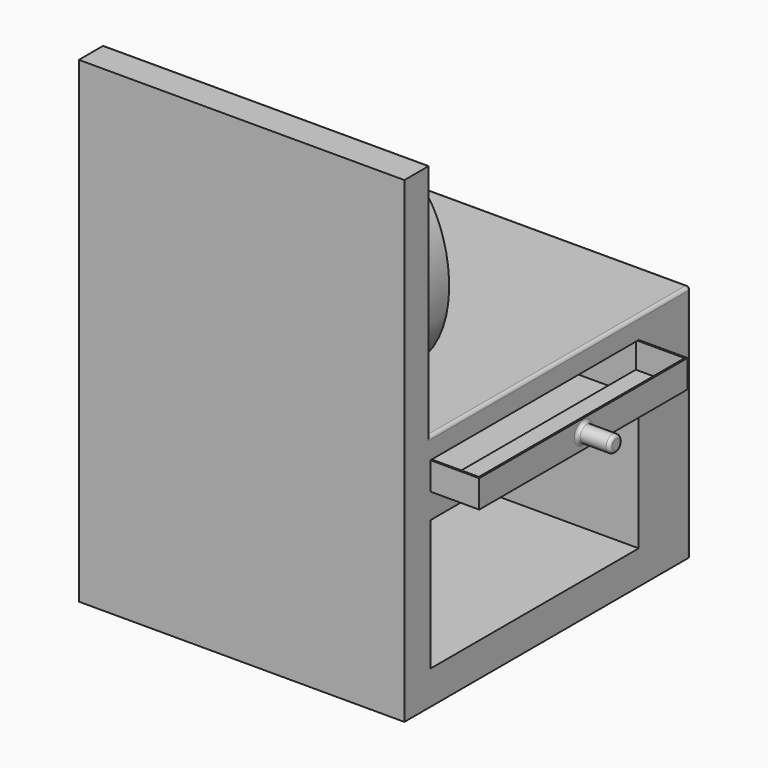
from build123d import *

# Parameters (mm, degrees)
F0_W         = 406.4
F0_H         = 203.9072960615
F1_DEPTH     = 508
F3_DEPTH     = 66.04
F4_W         = 101.6
F4_H         = 123.825
F5_DEPTH     = 88.9
F6_W         = 406.4
F6_H         = 43.1739762425
F7_DEPTH     = 76.2
F8_T         = 2.54
F8_T3_DEPTH  = 513.08
F8_T5_DEPTH  = 48.2539762425
F8_T7_DEPTH  = 411.48
F8_T9_DEPTH  = 93.98
F8_T11_DEPTH = 106.68
F8_T13_DEPTH = 128.905
F8_T15_DEPTH = 106.68
F8_T17_DEPTH = 106.68
F9_R         = 12.7
F10_DEPTH    = 50.8
F11_R        = 5.08


# Not quite as in the source:
# - a shell that OpenCascade refuses in one call is made with other operations: the cavity is built on its own and cut out


with BuildPart() as f1:
    # F0 (on Right) → F1 (new body)
    with BuildSketch(Plane.YZ):
        Polygon((-406.4, 487.9180668924), (-457.2, 487.9180668924), (-457.2, -256.5294758297), (-406.4, -256.5294758297), (0, -256.5294758297), (101.6, -256.5294758297), (101.6, 115.6942955313), (-406.4, 115.6942955313), align=None)
        with Locations((-203.2, -101.9536480308)):
            Rectangle(F0_W, F0_H, mode=Mode.SUBTRACT)
    extrude(amount=F1_DEPTH)

    # F4 (on face) → F5 (cut)
    with BuildSketch(Plane(origin=(0, 101.6, 0), x_dir=(-1, 0, 0), z_dir=(0, 1, 0))):
        with Locations((-434.9174816871, -150.9387567639)):
            Rectangle(F4_W, F4_H)
        with Locations((-258.955590483, -150.9387567639)):
            Rectangle(F4_W, F4_H)
        with Locations((-82.984390483, -150.9387567639)):
            Rectangle(F4_W, F4_H)
    extrude(amount=-F5_DEPTH, mode=Mode.SUBTRACT)

    # F6 (on face) → F7 (join)
    with BuildSketch(Plane.YZ.offset(508)):
        with Locations((-203.2, 60.8287490904)):
            Rectangle(F6_W, F6_H)
    extrude(amount=F7_DEPTH)

    # F8: shell of thickness 2.54, made by hand


with BuildPart() as f3:
    # F2 (on face) → F3 (new body)
    with BuildSketch(Plane(origin=(0, -406.4, 0), x_dir=(-1, 0, 0), z_dir=(0, 1, 0))):
        with BuildLine():
            add(Edge.make_bspline(
                [(-288.5718345642, 419.7029471397), (-347.6021943127, 419.1585833452), (-459.5465679813, 479.02511134), (-545.5014679601, 101.5749100376), (9.3815956545, 69.448257945), (-42.615563951, 501.5186421954), (-218.7578993917, 420.3467544759), (-288.5718345642, 419.7029471397)],
                knots=[0, 0, 0, 0, 0.1571960663, 0.3561031036, 0.6066974638, 0.8140875979, 1, 1, 1, 1], degree=3))
        make_face()
    extrude(amount=F3_DEPTH)


with BuildPart() as f8_core1:
    # F8_t2: copy of F1
    add(f1.part)

    # the walls: a layer under each face that stays
    f8_faces = [f8_core1.faces().sort_by_distance(p)[0] for p in [
        (254, -152.4, 115.6942955313),
        (254, 101.6, -70.4175901492),
        (254, -406.4, 301.8061812119),
        (0, 8.4666666667, -132.454885376),
        (508, 8.4666666667, -132.454885376),
        (254, -177.8, -256.5294758297),
        (258.955590483, 57.15, -212.8512567639),
        (309.755590483, 57.15, -150.9387567639),
        (258.955590483, 57.15, -89.0262567639),
        (208.155590483, 57.15, -150.9387567639),
        (485.7174816871, 57.15, -150.9387567639),
        (434.9174816871, 57.15, -89.0262567639),
        (384.1174816871, 57.15, -150.9387567639),
        (434.9174816871, 57.15, -212.8512567639),
        (82.984390483, 57.15, -212.8512567639),
        (133.784390483, 57.15, -150.9387567639),
        (82.984390483, 57.15, -89.0262567639),
        (32.184390483, 57.15, -150.9387567639),
        (254, -431.8, 487.9180668924),
        (254, -457.2, 115.6942955313),
        (254, -406.4, -101.9536480308),
        (254, -203.2, 0),
        (254, 0, -101.9536480308),
        (254, -203.2, -203.9072960615),
        (546.1, -406.4, 60.8287490904),
        (546.1, -203.2, 39.2417609692),
        (546.1, 0, 60.8287490904),
        (258.955590483, 12.7, -150.9387567639),
        (434.9174816871, 12.7, -150.9387567639),
        (82.984390483, 12.7, -150.9387567639),
        (584.2, -203.2, 60.8287490904),
    ]]
    thicken(f8_faces, amount=-F8_T, mode=Mode.SUBTRACT)

    # F8_s4 → F8_t3 (cut)
    with BuildSketch(Plane.YZ.offset(-2.54)):
        Polygon((-406.3746, 115.7196955313), (-406.4, 113.1542955313), (-408.94, 113.1542955313), (-408.94, 115.6942955313), align=None)
        Polygon((-406.3746, -203.8818960615), (-408.94, -203.9072960615), (-408.94, -206.4472960615), (-406.4, -206.4472960615), align=None)
        Polygon((-406.3746, -0.0254), (-408.94, 0), (-408.94, 2.54), (-406.4, 2.54), align=None)
        Polygon((-0.0254, -0.0254), (0, 2.54), (2.54, 2.54), (2.54, 0), align=None)
        Polygon((-0.0254, -203.8818960615), (2.54, -203.9072960615), (2.54, -206.4472960615), (0, -206.4472960615), align=None)
    extrude(amount=F8_T3_DEPTH, mode=Mode.SUBTRACT)

    # F8_s6 → F8_t5 (cut)
    with BuildSketch(Plane.XY.offset(36.7017609692)):
        Polygon((508.0254, -406.4254), (505.46, -406.4), (505.46, -403.86), (508, -403.86), align=None)
        Polygon((508.0254, 0.0254), (505.46, 0), (505.46, -2.54), (508, -2.54), align=None)
    extrude(amount=F8_T5_DEPTH, mode=Mode.SUBTRACT)

    # F8_s8 → F8_t7 (cut)
    with BuildSketch(Plane.XZ.offset(-2.54)):
        Polygon((508.0254, 39.2163609692), (505.46, 39.2417609692), (505.46, 41.7817609692), (508, 41.7817609692), align=None)
    extrude(amount=F8_T7_DEPTH, mode=Mode.SUBTRACT)

    # F8_s10 → F8_t9 (cut)
    with BuildSketch(Plane.XZ.offset(-104.14)):
        Polygon((309.730190483, -212.8258567639), (309.755590483, -215.3912567639), (312.295590483, -215.3912567639), (312.295590483, -212.8512567639), align=None)
        Polygon((208.180990483, -212.8258567639), (208.155590483, -215.3912567639), (205.615590483, -215.3912567639), (205.615590483, -212.8512567639), align=None)
        Polygon((309.730190483, -89.0516567639), (312.295590483, -89.0262567639), (312.295590483, -86.4862567639), (309.755590483, -86.4862567639), align=None)
        Polygon((208.180990483, -89.0516567639), (208.155590483, -86.4862567639), (205.615590483, -86.4862567639), (205.615590483, -89.0262567639), align=None)
        Polygon((485.6920816871, -89.0516567639), (488.2574816871, -89.0262567639), (488.2574816871, -86.4862567639), (485.7174816871, -86.4862567639), align=None)
        Polygon((485.6920816871, -212.8258567639), (488.2574816871, -212.8512567639), (488.2574816871, -215.3912567639), (485.7174816871, -215.3912567639), align=None)
        Polygon((384.1428816871, -89.0516567639), (384.1174816871, -86.4862567639), (381.5774816871, -86.4862567639), (381.5774816871, -89.0262567639), align=None)
        Polygon((384.1428816871, -212.8258567639), (381.5774816871, -212.8512567639), (381.5774816871, -215.3912567639), (384.1174816871, -215.3912567639), align=None)
        Polygon((133.758990483, -212.8258567639), (133.784390483, -215.3912567639), (136.324390483, -215.3912567639), (136.324390483, -212.8512567639), align=None)
        Polygon((32.209790483, -212.8258567639), (32.184390483, -215.3912567639), (29.644390483, -215.3912567639), (29.644390483, -212.8512567639), align=None)
        Polygon((133.758990483, -89.0516567639), (136.324390483, -89.0262567639), (136.324390483, -86.4862567639), (133.784390483, -86.4862567639), align=None)
        Polygon((32.209790483, -89.0516567639), (32.184390483, -86.4862567639), (29.644390483, -86.4862567639), (29.644390483, -89.0262567639), align=None)
    extrude(amount=F8_T9_DEPTH, mode=Mode.SUBTRACT)

    # F8_s12 → F8_t11 (cut)
    with BuildSketch(Plane.YZ.offset(205.615590483)):
        Polygon((12.7254, -212.8258567639), (12.7, -215.3912567639), (10.16, -215.3912567639), (10.16, -212.8512567639), align=None)
        Polygon((12.7254, -89.0516567639), (12.7, -86.4862567639), (10.16, -86.4862567639), (10.16, -89.0262567639), align=None)
    extrude(amount=F8_T11_DEPTH, mode=Mode.SUBTRACT)

    # F8_s14 → F8_t13 (cut)
    with BuildSketch(Plane.XY.offset(-215.3912567639)):
        Polygon((309.730190483, 12.7254), (312.295590483, 12.7), (312.295590483, 10.16), (309.755590483, 10.16), align=None)
        Polygon((208.180990483, 12.7254), (205.615590483, 12.7), (205.615590483, 10.16), (208.155590483, 10.16), align=None)
        Polygon((485.6920816871, 12.7254), (488.2574816871, 12.7), (488.2574816871, 10.16), (485.7174816871, 10.16), align=None)
        Polygon((384.1428816871, 12.7254), (381.5774816871, 12.7), (381.5774816871, 10.16), (384.1174816871, 10.16), align=None)
        Polygon((133.758990483, 12.7254), (136.324390483, 12.7), (136.324390483, 10.16), (133.784390483, 10.16), align=None)
        Polygon((32.209790483, 12.7254), (29.644390483, 12.7), (29.644390483, 10.16), (32.184390483, 10.16), align=None)
    extrude(amount=F8_T13_DEPTH, mode=Mode.SUBTRACT)

    # F8_s16 → F8_t15 (cut)
    with BuildSketch(Plane.YZ.offset(381.5774816871)):
        Polygon((12.7254, -89.0516567639), (12.7, -86.4862567639), (10.16, -86.4862567639), (10.16, -89.0262567639), align=None)
        Polygon((12.7254, -212.8258567639), (12.7, -215.3912567639), (10.16, -215.3912567639), (10.16, -212.8512567639), align=None)
    extrude(amount=F8_T15_DEPTH, mode=Mode.SUBTRACT)

    # F8_s18 → F8_t17 (cut)
    with BuildSketch(Plane.YZ.offset(29.644390483)):
        Polygon((12.7254, -212.8258567639), (12.7, -215.3912567639), (10.16, -215.3912567639), (10.16, -212.8512567639), align=None)
        Polygon((12.7254, -89.0516567639), (12.7, -86.4862567639), (10.16, -86.4862567639), (10.16, -89.0262567639), align=None)
    extrude(amount=F8_T17_DEPTH, mode=Mode.SUBTRACT)


with BuildPart() as f1_1:
    add(f1.part)

    # what is left inside the walls is the cavity
    f8_cavity = [f8_core1.part.solids().sort_by_distance(p)[0] for p in [
        (337.82, -454.6346, 115.694296),
    ]]
    add(f8_cavity, mode=Mode.SUBTRACT)

    # F9 (on face) → F10 (join)
    with BuildSketch(Plane.YZ.offset(584.2)):
        with Locations((-203.2, 62.6358613372)):
            Circle(F9_R)
    extrude(amount=F10_DEPTH)

    # F11
    f11_edges = [f1_1.edges().sort_by_distance(p)[0] for p in [
        (508, 101.6, -70.41759),
        (0, 101.6, -70.41759),
        (254, 101.6, 115.694296),
        (0, -152.4, 115.694296),
        (0, -406.4, 301.806181),
        (254, -406.4, 487.918067),
        (508, -406.4, 301.806181),
        (508, -152.4, 115.694296),
        (609.6, -190.5, 62.635861),
        (584.2, -215.9, 62.635861),
        (635, -215.9, 62.635861),
        (0, -406.4, -101.953648),
        (0, -203.2, 0),
        (0, 0, -101.953648),
        (0, -203.2, -203.907296),
    ]]
    fillet(f11_edges, radius=F11_R)


solid = Compound([f3.part, f1_1.part])
